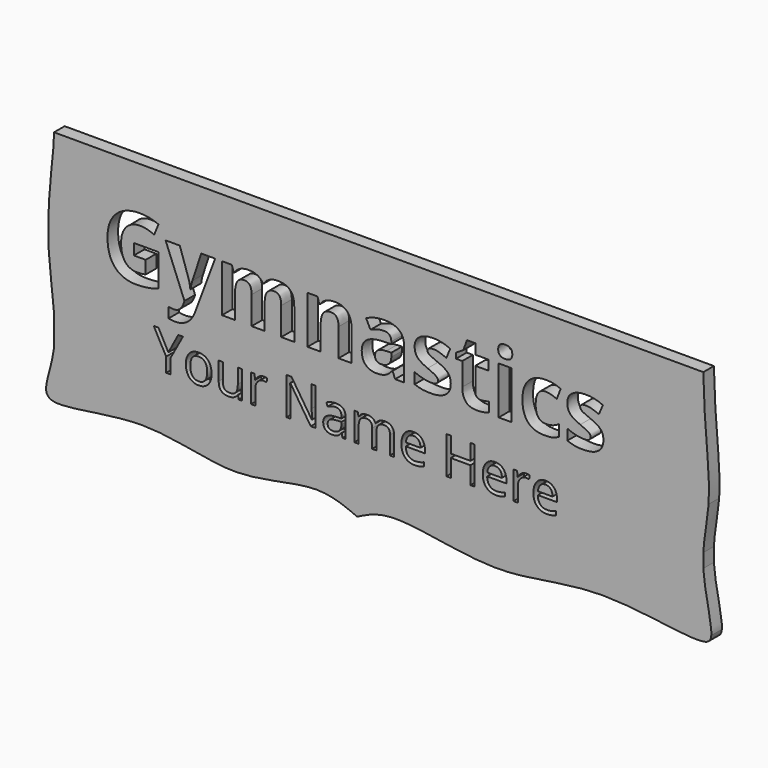
from build123d import *

# Parameters (mm, degrees)
F0_W         = 622.3
F0_H         = 219.71
F1_DEPTH     = 12.7
F2_TEXT_SIZE = 83.5725143433
F3_TEXT_SIZE = 50.0563092323
F4_DEPTH     = 25.4
F5_W         = 12.4444697139
F5_H         = 45.6253695493
F6_DEPTH     = 12.7


# Not quite as in the source:
# - Text() gives the source's letters only with a copy of the font that has no kerning and outlines rounded to 1/6400 em; it was checked with that copy


with BuildPart() as f1:
    # F0 (on Front) → F1 (new body)
    with BuildSketch(Plane.XZ):
        with Locations((20.5820777893, -3.9109852161)):
            Rectangle(F0_W, F0_H)
    extrude(amount=F1_DEPTH)

    # F2 (on face) + F3 (on face) → F4 (cut)
    with BuildSketch(Plane.XZ.offset(12.7)):
        with Locations((-244.2139566496, 3.9248836317)):
            Text('Gymnastics', F2_TEXT_SIZE, font='Open Sans', font_style=FontStyle.BOLD, text_align=(TextAlign.LEFT, TextAlign.BOTTOM))
    with BuildSketch(Plane.XZ.offset(12.7)):
        with Locations((-195.0602680445, -62.0602369308)):
            Text('Your Name Here', F3_TEXT_SIZE, font='Open Sans', text_align=(TextAlign.LEFT, TextAlign.BOTTOM))
    extrude(amount=-F4_DEPTH, mode=Mode.SUBTRACT)

    # F5 (on face) → F6 (join)
    with BuildSketch(Plane.XZ.offset(12.7)):
        with BuildLine():
            Line((0, -113.7659852161), (-38.9948076344, -113.7659852161))
            add(Edge.make_bspline(
                [(-38.9948076344, -113.7659852161), (-23.7077914674, -113.7998251226), (-11.8928807187, -118.8459366123), (0, -123.9259852161)],
                knots=[0.9046401261, 0.9046401261, 0.9046401261, 0.9046401261, 1, 1, 1, 1], degree=3))
            Line((0, -123.9259852161), (0, -113.7659852161))
        make_face()
        with BuildLine():
            Line((0, -113.7659852161), (0, -123.9259852161))
            add(Edge.make_bspline(
                [(33.4181897342, -113.7659852161), (18.7696313337, -114.397214566), (9.2754221357, -119.2324373573), (0, -123.9259852161)],
                knots=[0.9141845392, 0.9141845392, 0.9141845392, 0.9141845392, 1, 1, 1, 1], degree=3))
            Line((33.4181897343, -113.7659852161), (0, -113.7659852161))
        make_face()
        with BuildLine():
            Line((-115.3574213386, -113.7659852161), (-115.3574213386, -123.9259852161))
            add(Edge.make_bspline(
                [(-115.3574213386, -123.9259852161), (-88.4472145967, -123.5256265977), (-60.5272248515, -113.8129256595), (-39.3042191863, -113.7659852161)],
                knots=[0.7720146402, 0.7720146402, 0.7720146402, 0.7720146402, 0.9039977451, 0.9039977451, 0.9039977451, 0.9039977451], degree=3))
            Line((-39.3042191863, -113.7659852161), (-115.3574213386, -113.7659852161))
        make_face()
        with BuildLine():
            Line((-115.3574213386, -113.7659852161), (-205.5865424126, -113.7659852161))
            add(Edge.make_bspline(
                [(-205.5865424126, -113.7659852161), (-172.4059215865, -113.8913066112), (-144.4726963732, -124.3591499032), (-115.3574213386, -123.9259852161)],
                knots=[0.6292166144, 0.6292166144, 0.6292166144, 0.6292166144, 0.7720146402, 0.7720146402, 0.7720146402, 0.7720146402], degree=3))
            Line((-115.3574213386, -123.9259852161), (-115.3574213386, -113.7659852161))
        make_face()
        with BuildLine():
            Line((-206.7851424218, -113.7659852161), (-290.5679222107, -113.7659852161))
            Line((-290.5679222107, -113.7659852161), (-290.5679222107, -121.3859852161))
            add(Edge.make_bspline(
                [(-290.5679222107, -121.3859852161), (-276.2432745432, -123.9369942913), (-239.0205349915, -113.8882619563), (-206.7851424217, -113.7659852161)],
                knots=[0.4892995577, 0.4892995577, 0.4892995577, 0.4892995577, 0.6275004376, 0.6275004376, 0.6275004376, 0.6275004376], degree=3))
        make_face()
        with BuildLine():
            Line((-290.5679222107, -113.7659852161), (-298.1879222107, -113.7659852161))
            add(Edge.make_bspline(
                [(-298.1879222107, -113.7659852161), (-297.8884483653, -117.9460242514), (-295.6947312883, -120.4729759199), (-290.5679222107, -121.3859852161)],
                knots=[0.4398372922, 0.4398372922, 0.4398372922, 0.4398372922, 0.4892995577, 0.4892995577, 0.4892995577, 0.4892995577], degree=3))
            Line((-290.5679222107, -121.3859852161), (-290.5679222107, -113.7659852161))
        make_face()
        with BuildLine():
            Line((-290.5679222107, -113.7659852161), (-290.5679222107, -75.665985216))
            add(Edge.make_bspline(
                [(-290.5679222107, -75.6659852161), (-292.4954303089, -91.9313359206), (-298.7565718097, -105.8288062002), (-298.1879222107, -113.7659852161)],
                knots=[0.3459169119, 0.3459169119, 0.3459169119, 0.3459169119, 0.4398372922, 0.4398372922, 0.4398372922, 0.4398372922], degree=3))
            Line((-298.1879222107, -113.7659852161), (-290.5679222107, -113.7659852161))
        make_face()
        with BuildLine():
            Line((-290.5679222107, -46.9201377643), (-290.5679222107, 4.3440147839))
            Line((-290.5679222107, 4.3440147839), (-295.6479222107, 4.3440147839))
            add(Edge.make_bspline(
                [(-295.6479222107, 4.3440147839), (-294.6144050147, -13.1702112496), (-291.8699066313, -30.6290122267), (-290.5679222107, -46.9201377643)],
                knots=[0.2110057255, 0.2110057255, 0.2110057255, 0.2110057255, 0.2942177148, 0.2942177148, 0.2942177148, 0.2942177148], degree=3))
        make_face()
        with BuildLine():
            Line((-290.5679222107, 4.3440147839), (-290.5679222107, 74.1940147839))
            Line((-290.5679222107, 74.1940147839), (-293.1079222107, 74.1940147839))
            add(Edge.make_bspline(
                [(-293.1079222107, 74.1940147839), (-294.8560081938, 57.4984825083), (-297.212501225, 30.8577395787), (-295.6479222107, 4.3440147839)],
                knots=[0.0850361406, 0.0850361406, 0.0850361406, 0.0850361406, 0.2110057255, 0.2110057255, 0.2110057255, 0.2110057255], degree=3))
            Line((-295.6479222107, 4.3440147839), (-290.5679222107, 4.3440147839))
        make_face()
        with BuildLine():
            Line((-290.5679222107, 105.9440147839), (-290.5679222107, 74.1940147839))
            Line((-290.5679222107, 74.1940147839), (-290.5679222107, 4.3440147839))
            Line((-290.5679222107, 4.3440147839), (-290.5679222107, -46.9201377643))
            add(Edge.make_bspline(
                [(-290.5679222107, -46.9201377643), (-289.7590057341, -57.0417334302), (-289.5069105237, -66.7125975723), (-290.5679222107, -75.6659852161)],
                knots=[0.2942177148, 0.2942177148, 0.2942177148, 0.2942177148, 0.3459169119, 0.3459169119, 0.3459169119, 0.3459169119], degree=3))
            Line((-290.5679222107, -75.665985216), (-290.5679222107, -113.7659852161))
            Line((-290.5679222107, -113.7659852161), (-206.7851424218, -113.7659852161))
            add(Edge.make_bspline(
                [(-206.7851424217, -113.7659852161), (-206.3848437247, -113.764466785), (-205.9853141086, -113.7644790771), (-205.5865424126, -113.7659852161)],
                knots=[0.6275004376, 0.6275004376, 0.6275004376, 0.6275004376, 0.6292166144, 0.6292166144, 0.6292166144, 0.6292166144], degree=3))
            Line((-205.5865424126, -113.7659852161), (-115.3574213386, -113.7659852161))
            Line((-115.3574213386, -113.7659852161), (-39.3042191863, -113.7659852161))
            add(Edge.make_bspline(
                [(-39.3042191863, -113.7659852161), (-39.2009237185, -113.7657567501), (-39.0977868963, -113.7657572573), (-38.9948076344, -113.7659852161)],
                knots=[0.9039977451, 0.9039977451, 0.9039977451, 0.9039977451, 0.9046401261, 0.9046401261, 0.9046401261, 0.9046401261], degree=3))
            Line((-38.9948076344, -113.7659852161), (0, -113.7659852161))
            Line((0, -113.7659852161), (33.4181897343, -113.7659852161))
            add(Edge.make_bspline(
                [(40.8108736554, -113.7659852161), (38.2263464594, -113.671584288), (35.7565941218, -113.6652197045), (33.4181897342, -113.7659852161)],
                knots=[0.9004854949, 0.9004854949, 0.9004854949, 0.9004854949, 0.9141845392, 0.9141845392, 0.9141845392, 0.9141845392], degree=3))
            Line((40.8108736554, -113.7659852161), (131.6767185926, -113.7659852161))
            Line((131.6767185926, -113.7659852161), (234.9624951182, -113.7659852161))
            add(Edge.make_bspline(
                [(235.4865521193, -113.7659852161), (235.3117017675, -113.7657620078), (235.1370165153, -113.7657627033), (234.9624951182, -113.7659852161)],
                knots=[0.6215721476, 0.6215721476, 0.6215721476, 0.6215721476, 0.6222517313, 0.6222517313, 0.6222517313, 0.6222517313], degree=3))
            Line((235.4865521193, -113.7659852161), (331.7320777893, -113.7659852161))
            Line((331.7320777893, -113.7659852161), (331.7320777893, -59.7018413246))
            add(Edge.make_bspline(
                [(331.7320777893, -46.2929872824), (331.4882954863, -50.6263940713), (331.4498437355, -55.0775546721), (331.7320777893, -59.7018413246)],
                knots=[0.2992799759, 0.2992799759, 0.2992799759, 0.2992799759, 0.3239405291, 0.3239405291, 0.3239405291, 0.3239405291], degree=3))
            Line((331.7320777893, -46.2929872824), (331.7320777893, -3.9109852161))
            Line((331.7320777893, -3.9109852161), (331.7320777893, 54.1004016995))
            Line((331.7320777893, 54.1004016995), (331.7320777893, 105.9440147839))
            Line((331.7320777893, 105.9440147839), (-290.5679222107, 105.9440147839))
        make_face()
        Polygon((-190.516093722, -26.324724918), (-181.0523227578, -44.1963915736), (-171.525981407, -26.324724918), (-167.0287348744, -26.324724918), (-178.9562148086, -48.2008963122), (-178.9562148086, -62.0602369308), (-183.1562520052, -62.0602369308), (-183.1562520052, -48.3964287701), (-195.0602680445, -26.324724918), align=None, mode=Mode.SUBTRACT)
        with BuildLine():
            add(Edge.make_bspline(
                [(-139.6072629731, -48.6388890179), (-139.6072629731, -42.2645308891), (-146.231902648, -34.7795483993), (-157.6666407883, -34.7795483993), (-164.2208887784, -42.0924623262), (-164.2208887784, -52.8702114077), (-161.1862250312, -59.1741778517), (-155.6174606291, -62.5529787249), (-146.2006174548, -62.5529787249), (-139.6072629731, -55.193137008), (-139.6072629731, -48.6388890179)],
                knots=[0, 0, 0, 1, 2, 3.0362116992, 4.0724233983, 4.742185082, 5.4119467657, 6.0817084494, 7.1649751726, 8.2482418958, 8.2482418958, 8.2482418958], degree=2))
        make_face(mode=Mode.SUBTRACT)
        with BuildLine():
            Line((-132.7792695419, -35.2722901933), (-128.6730879252, -35.2722901933))
            Line((-128.6730879252, -35.2722901933), (-128.6730879252, -52.6512150548))
            add(Edge.make_bspline(
                [(-114.4305036889, -49.3506271648), (-114.4305036889, -54.5596118443), (-118.3098676544, -59.1507139567), (-125.6931732662, -59.1507139567), (-128.6730879252, -55.9283390499), (-128.6730879252, -52.6512150548)],
                knots=[0, 0, 0, 1, 2, 2.7546468401, 3.5092936803, 3.5092936803, 3.5092936803], degree=2))
            Line((-114.4305036889, -49.3506271648), (-114.4305036889, -35.2722901933))
            Line((-114.4305036889, -35.2722901933), (-110.3712498621, -35.2722901933))
            Line((-110.3712498621, -35.2722901933), (-110.3712498621, -62.0602369308))
            Line((-110.3712498621, -62.0602369308), (-113.718765542, -62.0602369308))
            Line((-113.718765542, -62.0602369308), (-114.3053629158, -58.4702610031))
            Line((-114.3053629158, -58.4702610031), (-114.5243592687, -58.4702610031))
            add(Edge.make_bspline(
                [(-132.7792695419, -52.7998197229), (-132.7792695419, -57.9071275242), (-127.9222432867, -62.5529787249), (-120.1948005489, -62.5529787249), (-115.7679457012, -60.4490494774), (-114.5243592687, -58.4702610031)],
                knots=[0, 0, 0, 1, 2, 2.5808, 3.1616, 3.1616, 3.1616], degree=2))
            Line((-132.7792695419, -52.7998197229), (-132.7792695419, -35.2722901933))
        make_face(mode=Mode.SUBTRACT)
        with BuildLine():
            add(Edge.make_bspline(
                [(-86.3442214306, -35.0767577353), (-87.7598764261, -34.7795483993), (-92.0615905007, -34.7795483993), (-96.2694489956, -37.6186796885), (-97.7554956759, -40.2309933266)],
                knots=[0, 0, 0, 1, 2.4122807018, 3.8245614035, 3.8245614035, 3.8245614035], degree=2))
            Line((-86.3442214306, -35.0767577353), (-86.9073549095, -38.8388022261))
            add(Edge.make_bspline(
                [(-97.708567886, -47.6846906232), (-97.708567886, -43.7505775695), (-93.0940018787, -38.4712012051), (-88.5654701528, -38.4712012051), (-86.9073549095, -38.8388022261)],
                knots=[0, 0, 0, 1, 2, 2.3918269231, 2.3918269231, 2.3918269231], degree=2))
            Line((-97.708567886, -47.6846906232), (-97.708567886, -62.0602369308))
            Line((-97.708567886, -62.0602369308), (-101.7678217128, -62.0602369308))
            Line((-101.7678217128, -62.0602369308), (-101.7678217128, -35.2722901933))
            Line((-101.7678217128, -35.2722901933), (-98.4203060329, -35.2722901933))
            Line((-98.4203060329, -35.2722901933), (-97.9510281338, -40.2309933266))
            Line((-97.9510281338, -40.2309933266), (-97.7554956759, -40.2309933266))
        make_face(mode=Mode.SUBTRACT)
        with BuildLine():
            Line((-11.1033316158, -62.0602369308), (-14.1145314681, -62.0602369308))
            Line((-14.1145314681, -62.0602369308), (-14.9201251948, -58.2434433519))
            Line((-14.9201251948, -58.2434433519), (-15.1156576527, -58.2434433519))
            add(Edge.make_bspline(
                [(-19.6129041853, -46.151716153), (-32.5884380941, -46.5427810688), (-32.5884380941, -58.4389758098), (-28.0677276666, -62.5529787249), (-21.0989508657, -62.5529787249), (-17.117910022, -60.7619014101), (-15.1156576527, -58.2434433519)],
                knots=[0, 0, 0, 1, 1.4667309547, 1.9334619094, 2.2837393645, 2.6340168197, 2.6340168197, 2.6340168197], degree=2))
            Line((-19.6129041853, -46.151716153), (-15.0687298628, -46.0031114849))
            Line((-15.0687298628, -46.0031114849), (-15.0687298628, -44.3371749433))
            add(Edge.make_bspline(
                [(-28.3336518094, -40.2309933266), (-24.1101507179, -38.1818131674), (-17.7748990807, -38.1818131674), (-15.0687298628, -41.1851917213), (-15.0687298628, -44.3371749433)],
                knots=[0, 0, 0, 1, 1.8925233645, 2.785046729, 2.785046729, 2.785046729], degree=2))
            Line((-28.3336518094, -40.2309933266), (-29.5850595402, -37.1259378945))
            add(Edge.make_bspline(
                [(-11.1033316158, -43.7740414644), (-11.1033316158, -39.0812624739), (-15.7257189215, -34.8342974875), (-22.8900281804, -34.8342974875), (-27.6062710659, -36.054420025), (-29.5850595402, -37.1259378945)],
                knots=[0, 0, 0, 1, 2, 2.4967320261, 2.9934640523, 2.9934640523, 2.9934640523], degree=2))
            Line((-11.1033316158, -43.7740414644), (-11.1033316158, -62.0602369308))
        make_face(mode=Mode.SUBTRACT)
        with BuildLine():
            Line((-67.7138888382, -26.324724918), (-63.0211098477, -26.324724918))
            Line((-63.0211098477, -26.324724918), (-43.5382557387, -56.1942631927))
            Line((-43.5382557387, -56.1942631927), (-43.3427232808, -56.1942631927))
            add(Edge.make_bspline(
                [(-43.6868604067, -46.8321691066), (-43.7337881966, -48.3729648751), (-43.3896510707, -55.537274134), (-43.3427232808, -56.1942631927)],
                knots=[0, 0, 0, 1, 2, 2, 2], degree=2))
            Line((-43.6868604067, -46.8321691066), (-43.6868604067, -26.324724918))
            Line((-43.6868604067, -26.324724918), (-39.7996751429, -26.324724918))
            Line((-39.7996751429, -26.324724918), (-39.7996751429, -62.0602369308))
            Line((-39.7996751429, -62.0602369308), (-44.5393819233, -62.0602369308))
            Line((-44.5393819233, -62.0602369308), (-64.0691638222, -32.0733791814))
            Line((-64.0691638222, -32.0733791814), (-64.2646962802, -32.0733791814))
            add(Edge.make_bspline(
                [(-64.2646962802, -32.0733791814), (-63.8736313643, -37.3527555457), (-63.8736313643, -41.7483252002)],
                knots=[0, 0, 0, 1, 1, 1], degree=2))
            Line((-63.8736313643, -41.7483252002), (-63.8736313643, -62.0602369308))
            Line((-63.8736313643, -62.0602369308), (-67.7138888382, -62.0602369308))
            Line((-67.7138888382, -62.0602369308), (-67.7138888382, -26.324724918))
        make_face(mode=Mode.SUBTRACT)
        with BuildLine():
            Line((35.4490359702, -62.0602369308), (31.3976034417, -62.0602369308))
            Line((31.3976034417, -62.0602369308), (31.3976034417, -44.6343842794))
            add(Edge.make_bspline(
                [(18.3673204447, -47.0980932494), (18.3673204447, -42.5773828218), (21.9885815657, -38.2287409573), (28.6601490306, -38.2287409573), (31.3976034417, -41.4276519692), (31.3976034417, -44.6343842794)],
                knots=[0, 0, 0, 1, 2, 2.7623966942, 3.5247933884, 3.5247933884, 3.5247933884], degree=2))
            Line((18.3673204447, -47.0980932494), (18.3673204447, -62.0602369308))
            Line((18.3673204447, -62.0602369308), (14.3080666179, -62.0602369308))
            Line((14.3080666179, -62.0602369308), (14.3080666179, -44.6343842794))
            add(Edge.make_bspline(
                [(1.3090688141, -48.0053638542), (1.3090688141, -42.7963791747), (4.852116952, -38.2287409573), (11.5706122067, -38.2287409573), (14.3080666179, -41.4276519692), (14.3080666179, -44.6343842794)],
                knots=[0, 0, 0, 1, 2, 2.7638603696, 3.5277207392, 3.5277207392, 3.5277207392], degree=2))
            Line((1.3090688141, -48.0053638542), (1.3090688141, -62.0602369308))
            Line((1.3090688141, -62.0602369308), (-2.7501850127, -62.0602369308))
            Line((-2.7501850127, -62.0602369308), (-2.7501850127, -35.2722901933))
            Line((-2.7501850127, -35.2722901933), (0.5504028773, -35.2722901933))
            Line((0.5504028773, -35.2722901933), (1.207391936, -38.9404791042))
            Line((1.207391936, -38.9404791042), (1.4029243939, -38.9404791042))
            add(Edge.make_bspline(
                [(17.538262823, -39.3315440201), (15.6064021386, -34.7795483993), (6.7370498465, -34.7795483993), (2.5526552466, -36.9851545248), (1.4029243939, -38.9404791042)],
                knots=[0, 0, 0, 1, 1.4122042341, 1.8244084682, 1.8244084682, 1.8244084682], degree=2))
            Line((17.538262823, -39.3315440201), (17.7337952809, -39.3315440201))
            add(Edge.make_bspline(
                [(35.4490359702, -44.5874564895), (35.4490359702, -39.4488634948), (30.9283255426, -34.7795483993), (23.474628246, -34.7795483993), (18.9304539235, -37.2276147726), (17.7337952809, -39.3315440201)],
                knots=[0, 0, 0, 1, 2, 2.6402753873, 3.2805507745, 3.2805507745, 3.2805507745], degree=2))
            Line((35.4490359702, -44.5874564895), (35.4490359702, -62.0602369308))
        make_face(mode=Mode.SUBTRACT)
        with BuildLine():
            add(Edge.make_bspline(
                [(64.9744371189, -46.8321691066), (64.9744371189, -41.4041880742), (59.1084633808, -34.7795483993), (48.6983153201, -34.7795483993), (42.316135893, -42.4053142589), (42.316135893, -55.3104564828), (49.1910571141, -62.5529787249), (57.8414130533, -62.5529787249), (61.6738492289, -61.7395636998), (63.8247062662, -60.8166504984)],
                knots=[0, 0, 0, 1, 2, 3.0699844479, 4.1399688958, 5.1996278002, 6.2592867045, 6.743742093, 7.2281974814, 7.2281974814, 7.2281974814], degree=2))
            Line((64.9744371189, -46.8321691066), (64.9744371189, -49.3975549547))
            Line((64.9744371189, -49.3975549547), (46.5239943878, -49.3975549547))
            add(Edge.make_bspline(
                [(63.8247062662, -57.1953893773), (59.6012051748, -59.0021092887), (51.1698455884, -59.0021092887), (46.6491351609, -54.1137978402), (46.5239943878, -49.3975549547)],
                knots=[0, 0, 0, 1, 1.9493670886, 2.8987341772, 2.8987341772, 2.8987341772], degree=2))
            Line((63.8247062662, -57.1953893773), (63.8247062662, -60.8166504984))
        make_face(mode=Mode.SUBTRACT)
        Polygon((112.6452503643, -26.324724918), (112.6452503643, -62.0602369308), (108.4921409577, -62.0602369308), (108.4921409577, -45.2444455481), (89.6662759074, -45.2444455481), (89.6662759074, -62.0602369308), (85.5131665008, -62.0602369308), (85.5131665008, -26.324724918), (89.6662759074, -26.324724918), (89.6662759074, -41.5293288473), (108.4921409577, -41.5293288473), (108.4921409577, -26.324724918), align=None, mode=Mode.SUBTRACT)
        with BuildLine():
            add(Edge.make_bspline(
                [(142.9997091347, -46.8321691066), (142.9997091347, -41.4041880742), (137.1337353966, -34.7795483993), (126.7235873359, -34.7795483993), (120.3414079088, -42.4053142589), (120.3414079088, -55.3104564828), (127.2163291299, -62.5529787249), (135.8666850691, -62.5529787249), (139.6991212447, -61.7395636998), (141.8499782821, -60.8166504984)],
                knots=[0, 0, 0, 1, 2, 3.0699844479, 4.1399688958, 5.1996278002, 6.2592867045, 6.743742093, 7.2281974814, 7.2281974814, 7.2281974814], degree=2))
            Line((142.9997091347, -46.8321691066), (142.9997091347, -49.3975549547))
            Line((142.9997091347, -49.3975549547), (124.5492664036, -49.3975549547))
            add(Edge.make_bspline(
                [(141.8499782821, -57.1953893773), (137.6264771906, -59.0021092887), (129.1951176043, -59.0021092887), (124.6744071767, -54.1137978402), (124.5492664036, -49.3975549547)],
                knots=[0, 0, 0, 1, 1.9493670886, 2.8987341772, 2.8987341772, 2.8987341772], degree=2))
            Line((141.8499782821, -57.1953893773), (141.8499782821, -60.8166504984))
        make_face(mode=Mode.SUBTRACT)
        with BuildLine():
            add(Edge.make_bspline(
                [(165.345158428, -35.0767577353), (163.9295034325, -34.7795483993), (159.6277893578, -34.7795483993), (155.419930863, -37.6186796885), (153.9338841827, -40.2309933266)],
                knots=[0, 0, 0, 1, 2.4122807018, 3.8245614035, 3.8245614035, 3.8245614035], degree=2))
            Line((165.345158428, -35.0767577353), (164.7820249491, -38.8388022261))
            add(Edge.make_bspline(
                [(153.9808119726, -47.6846906232), (153.9808119726, -43.7505775695), (158.5953779799, -38.4712012051), (163.1239097058, -38.4712012051), (164.7820249491, -38.8388022261)],
                knots=[0, 0, 0, 1, 2, 2.3918269231, 2.3918269231, 2.3918269231], degree=2))
            Line((153.9808119726, -47.6846906232), (153.9808119726, -62.0602369308))
            Line((153.9808119726, -62.0602369308), (149.9215581458, -62.0602369308))
            Line((149.9215581458, -62.0602369308), (149.9215581458, -35.2722901933))
            Line((149.9215581458, -35.2722901933), (153.2690738257, -35.2722901933))
            Line((153.2690738257, -35.2722901933), (153.7383517247, -40.2309933266))
            Line((153.7383517247, -40.2309933266), (153.9338841827, -40.2309933266))
        make_face(mode=Mode.SUBTRACT)
        with BuildLine():
            add(Edge.make_bspline(
                [(191.5230438968, -46.8321691066), (191.5230438968, -41.4041880742), (185.6570701586, -34.7795483993), (175.246922098, -34.7795483993), (168.8647426708, -42.4053142589), (168.8647426708, -55.3104564828), (175.739663892, -62.5529787249), (184.3900198312, -62.5529787249), (188.2224560068, -61.7395636998), (190.3733130441, -60.8166504984)],
                knots=[0, 0, 0, 1, 2, 3.0699844479, 4.1399688958, 5.1996278002, 6.2592867045, 6.743742093, 7.2281974814, 7.2281974814, 7.2281974814], degree=2))
            Line((191.5230438968, -46.8321691066), (191.5230438968, -49.3975549547))
            Line((191.5230438968, -49.3975549547), (173.0726011657, -49.3975549547))
            add(Edge.make_bspline(
                [(190.3733130441, -57.1953893773), (186.1498119526, -59.0021092887), (177.7184523663, -59.0021092887), (173.1977419388, -54.1137978402), (173.0726011657, -49.3975549547)],
                knots=[0, 0, 0, 1, 1.9493670886, 2.8987341772, 2.8987341772, 2.8987341772], degree=2))
            Line((190.3733130441, -57.1953893773), (190.3733130441, -60.8166504984))
        make_face(mode=Mode.SUBTRACT)
        with BuildLine():
            Line((-149.502793129, 49.550253181), (-136.1573072448, 49.550253181))
            Line((-136.1573072448, 49.550253181), (-155.457334776, -1.9121341669))
            add(Edge.make_bspline(
                [(-180.8424860078, -15.4534931316), (-177.747691336, -16.1586362214), (-167.9540373114, -16.1586362214), (-158.1212086707, -9.0549725022), (-155.457334776, -1.9121341669)],
                knots=[0, 0, 0, 1, 3.036437247, 5.0728744939, 5.0728744939, 5.0728744939], degree=2))
            Line((-180.8424860078, -15.4534931316), (-180.8424860078, -5.5814898748))
            add(Edge.make_bspline(
                [(-166.3217616406, 2.0053274429), (-167.7059314094, -2.0688326313), (-172.6419330378, -6.1168762948), (-178.5964746848, -6.1168762948), (-180.8424860078, -5.5814898748)],
                knots=[0, 0, 0, 1, 2, 2.8023715415, 2.8023715415, 2.8023715415], degree=2))
            Line((-166.3217616406, 2.0053274429), (-165.5774439347, 4.2513387659))
            Line((-165.5774439347, 4.2513387659), (-183.7022329829, 49.550253181))
            Line((-183.7022329829, 49.550253181), (-170.0694665807, 49.550253181))
            Line((-170.0694665807, 49.550253181), (-161.4641092444, 23.8778214312))
            add(Edge.make_bspline(
                [(-161.4641092444, 23.8778214312), (-160.3541617883, 20.5349208575), (-159.9493574219, 15.9645489793)],
                knots=[0, 0, 0, 1, 1, 1], degree=2))
            Line((-159.9493574219, 15.9645489793), (-159.70125152, 15.9645489793))
            add(Edge.make_bspline(
                [(-159.70125152, 15.9645489793), (-159.2572725375, 20.1692911072), (-157.9514520009, 23.8778214312)],
                knots=[0, 0, 0, 1, 1, 1], degree=2))
            Line((-157.9514520009, 23.8778214312), (-149.502793129, 49.550253181))
        make_face(mode=Mode.SUBTRACT)
        with BuildLine():
            Line((-214.0625604592, 37.4322386012), (-190.3880341304, 37.4322386012))
            Line((-190.3880341304, 37.4322386012), (-190.3880341304, 6.4973500889))
            add(Edge.make_bspline(
                [(-190.4663833626, 60.7672515905), (-198.9933914667, 64.4366072984), (-222.8246162599, 64.4366072984), (-239.3563042534, 48.2836072605), (-239.3563042534, 18.9809944189), (-225.109802199, 3.1022166937), (-206.3059864717, 3.1022166937), (-196.1467026969, 4.6169685161), (-190.3880341304, 6.4973500889)],
                knots=[0, 0, 0, 1, 2.5923295455, 4.1846590909, 5.823059654, 7.461460217, 8.1047780396, 8.7480958623, 8.7480958623, 8.7480958623], degree=2))
            Line((-190.4663833626, 60.7672515905), (-194.6711254905, 50.6471424318))
            add(Edge.make_bspline(
                [(-202.7541546121, 14.4497971568), (-206.8283146864, 13.6401884241), (-218.3848264354, 13.6401884241), (-226.3372735034, 23.8778214312), (-226.3372735034, 42.8905684443), (-216.4652702466, 53.9116937733), (-201.2002281736, 53.9116937733), (-194.6711254905, 50.6471424318)],
                knots=[0, 0, 0, 1, 2.9111842105, 4.8223684211, 6.6513511602, 8.4803338993, 10.0559384564, 10.0559384564, 10.0559384564], degree=2))
            Line((-202.7541546121, 14.4497971568), (-202.7541546121, 26.8942668708))
            Line((-202.7541546121, 26.8942668708), (-214.0625604592, 26.8942668708))
            Line((-214.0625604592, 26.8942668708), (-214.0625604592, 37.4322386012))
        make_face(mode=Mode.SUBTRACT)
        with BuildLine():
            add(Edge.make_bspline(
                [(-117.1837348478, 25.3925732537), (-117.1837348478, 33.4233695538), (-112.8614688717, 40.4486840408), (-104.5303338481, 40.4486840408), (-101.2266078904, 35.5126824124), (-101.2266078904, 30.576680784)],
                knots=[0, 0, 0, 1, 2, 2.7431693989, 3.4863387978, 3.4863387978, 3.4863387978], degree=2))
            Line((-117.1837348478, 25.3925732537), (-117.1837348478, 3.9248836317))
            Line((-117.1837348478, 3.9248836317), (-129.6282045618, 3.9248836317))
            Line((-129.6282045618, 3.9248836317), (-129.6282045618, 49.550253181))
            Line((-129.6282045618, 49.550253181), (-120.1218310552, 49.550253181))
            Line((-120.1218310552, 49.550253181), (-118.4503807684, 43.7132353824))
            Line((-118.4503807684, 43.7132353824), (-117.758295884, 43.7132353824))
            add(Edge.make_bspline(
                [(-90.6102869278, 43.7132353824), (-94.2535262249, 50.3990365298), (-108.9831818779, 50.3990365298), (-115.9170889273, 46.8602628756), (-117.758295884, 43.7132353824)],
                knots=[0, 0, 0, 1, 1.4387755102, 1.8775510204, 1.8775510204, 1.8775510204], degree=2))
            Line((-90.6102869278, 43.7132353824), (-89.513397677, 43.7132353824))
            add(Edge.make_bspline(
                [(-60.3413668891, 33.6714754558), (-60.3413668891, 42.4465894618), (-68.293813957, 50.3990365298), (-80.5424105905, 50.3990365298), (-87.6721907204, 46.8994374917), (-89.513397677, 43.7132353824)],
                knots=[0, 0, 0, 1, 2, 2.5791245791, 3.1582491582, 3.1582491582, 3.1582491582], degree=2))
            Line((-60.3413668891, 33.6714754558), (-60.3413668891, 3.9248836317))
            Line((-60.3413668891, 3.9248836317), (-72.8250112191, 3.9248836317))
            Line((-72.8250112191, 3.9248836317), (-72.8250112191, 30.576680784))
            add(Edge.make_bspline(
                [(-88.7821381765, 26.8159176386), (-88.7821381765, 33.9195813578), (-84.2509409145, 40.4486840408), (-76.1287371767, 40.4486840408), (-72.8250112191, 35.5126824124), (-72.8250112191, 30.576680784)],
                knots=[0, 0, 0, 1, 2, 2.7771428571, 3.5542857143, 3.5542857143, 3.5542857143], degree=2))
            Line((-88.7821381765, 26.8159176386), (-88.7821381765, 3.9248836317))
            Line((-88.7821381765, 3.9248836317), (-101.2266078904, 3.9248836317))
            Line((-101.2266078904, 3.9248836317), (-101.2266078904, 30.576680784))
        make_face(mode=Mode.SUBTRACT)
        with BuildLine():
            Line((-5.4577297352, 3.9248836317), (-17.9021994491, 3.9248836317))
            Line((-17.9021994491, 3.9248836317), (-17.9021994491, 30.576680784))
            add(Edge.make_bspline(
                [(-35.125972327, 25.3925732537), (-35.125972327, 33.4756023753), (-30.4772512167, 40.4486840408), (-21.4148566926, 40.4486840408), (-17.9021994491, 35.5126824124), (-17.9021994491, 30.576680784)],
                knots=[0, 0, 0, 1, 2, 2.735, 3.47, 3.47, 3.47], degree=2))
            Line((-35.125972327, 25.3925732537), (-35.125972327, 3.9248836317))
            Line((-35.125972327, 3.9248836317), (-47.570442041, 3.9248836317))
            Line((-47.570442041, 3.9248836317), (-47.570442041, 49.550253181))
            Line((-47.570442041, 49.550253181), (-38.0640685344, 49.550253181))
            Line((-38.0640685344, 49.550253181), (-36.3926182476, 43.7132353824))
            Line((-36.3926182476, 43.7132353824), (-35.7005333632, 43.7132353824))
            add(Edge.make_bspline(
                [(-5.4577297352, 33.6714754558), (-5.4577297352, 41.7936791935), (-13.6974573212, 50.3990365298), (-26.3116837049, 50.3990365298), (-33.6112205046, 47.01696134), (-35.7005333632, 43.7132353824)],
                knots=[0, 0, 0, 1, 2, 2.5836065574, 3.1672131148, 3.1672131148, 3.1672131148], degree=2))
            Line((-5.4577297352, 33.6714754558), (-5.4577297352, 3.9248836317))
        make_face(mode=Mode.SUBTRACT)
        with BuildLine():
            Line((36.3285274364, 3.9248836317), (33.9127594437, 10.1275311807))
            Line((33.9127594437, 10.1275311807), (33.5863043096, 10.1275311807))
            add(Edge.make_bspline(
                [(24.7328410713, 32.0783744011), (14.4952080643, 31.7127446509), (4.3359242894, 24.8180122176), (4.3359242894, 10.6237429846), (11.883566991, 3.1022166937), (23.792650285, 3.1022166937), (30.4523350217, 6.1708949547), (33.5863043096, 10.1275311807)],
                knots=[0, 0, 0, 1, 2, 2.9550359712, 3.9100719424, 4.6866320065, 5.4631920706, 5.4631920706, 5.4631920706], degree=2))
            Line((24.7328410713, 32.0783744011), (32.6591717286, 32.3264803031))
            Line((32.6591717286, 32.3264803031), (32.6591717286, 34.3243857241))
            add(Edge.make_bspline(
                [(12.6931757237, 37.9545668159), (20.084119961, 41.2582927735), (32.6591717286, 41.2582927735), (32.6591717286, 34.3243857241)],
                knots=[0, 0, 0, 1, 2.2983293556, 2.2983293556, 2.2983293556], degree=2))
            Line((12.6931757237, 37.9545668159), (8.5798410334, 46.3640510717))
            add(Edge.make_bspline(
                [(45.0122340049, 34.3243857241), (45.0122340049, 42.4857640779), (35.2185799803, 50.4904439674), (16.4539388692, 50.4904439674), (8.5798410334, 46.3640510717)],
                knots=[0, 0, 0, 1, 2, 3.0440967283, 3.0440967283, 3.0440967283], degree=2))
            Line((45.0122340049, 34.3243857241), (45.0122340049, 3.9248836317))
            Line((45.0122340049, 3.9248836317), (36.3285274364, 3.9248836317))
        make_face(mode=Mode.SUBTRACT)
        with BuildLine():
            add(Edge.make_bspline(
                [(55.145401369, 5.7660905884), (58.2010214247, 4.4602700518), (65.2263359117, 3.1022166937), (79.9168169486, 3.1022166937), (89.6712963571, 10.4539863148), (89.6712963571, 20.8613759916), (87.2947029805, 25.7582030039), (82.319526736, 29.505907944), (76.9787207412, 31.6735700348)],
                knots=[0, 0, 0, 1, 2, 3.9527559055, 5.905511811, 6.8455931856, 7.7856745602, 8.7257559348, 8.7257559348, 8.7257559348], degree=2))
            Line((55.145401369, 5.7660905884), (55.145401369, 16.0428982115))
            add(Edge.make_bspline(
                [(67.5115218508, 23.3032603951), (71.1808775587, 21.7623921619), (75.581492767, 19.4380316067), (77.3835251076, 17.5968246501), (77.3835251076, 12.2037858339), (67.3025905649, 12.2037858339), (58.6058257911, 14.4106225408), (55.145401369, 16.0428982115)],
                knots=[0, 0, 0, 1, 2, 3, 5.6548672566, 6.9490511024, 8.2432349481, 8.2432349481, 8.2432349481], degree=2))
            add(Edge.make_bspline(
                [(89.1750845532, 46.8080300541), (81.3793359496, 50.3990365298), (64.4820182058, 50.3990365298), (55.0670521368, 43.7524099985), (55.0670521368, 34.1285126436), (57.3000052545, 29.2708602474), (62.2490650882, 25.510097102), (67.5115218508, 23.3032603951)],
                knots=[0, 0, 0, 1, 2.0507131537, 3.1014263074, 3.7124633561, 4.3235004047, 4.9345374533, 4.9345374533, 4.9345374533], degree=2))
            Line((89.1750845532, 46.8080300541), (85.4273796131, 37.8370429676))
            add(Edge.make_bspline(
                [(76.9787207412, 31.6735700348), (70.9719462728, 34.0762798222), (67.4201144132, 36.531222431), (67.4201144132, 41.1799435413), (76.0385299549, 41.1799435413), (81.9930716018, 39.2995619686), (85.4273796131, 37.8370429676)],
                knots=[0, 0, 0, 1, 2, 3.78125, 4.7858412322, 5.7904324645, 5.7904324645, 5.7904324645], degree=2))
        make_face(mode=Mode.SUBTRACT)
        with BuildLine():
            add(Edge.make_bspline(
                [(126.4301444628, 14.4497971568), (121.8597725846, 13.0264527719), (116.1402786343, 13.0264527719), (113.1630078108, 15.559744613), (113.1630078108, 18.2105603023)],
                knots=[0, 0, 0, 1, 1.752, 2.504, 2.504, 2.504], degree=2))
            Line((126.4301444628, 14.4497971568), (126.4301444628, 5.1915295523))
            add(Edge.make_bspline(
                [(100.7185380969, 18.2105603023), (100.7185380969, 10.6629176007), (107.534921298, 3.1022166937), (121.7814233524, 3.1022166937), (126.4301444628, 5.1915295523)],
                knots=[0, 0, 0, 1, 2, 2.9073426573, 2.9073426573, 2.9073426573], degree=2))
            Line((100.7185380969, 18.2105603023), (100.7185380969, 40.2005781389))
            Line((100.7185380969, 40.2005781389), (94.7639964499, 40.2005781389))
            Line((94.7639964499, 40.2005781389), (94.7639964499, 45.4630349014))
            Line((94.7639964499, 45.4630349014), (101.6195542671, 49.6286024132))
            Line((101.6195542671, 49.6286024132), (105.2105607428, 59.2655579734))
            Line((105.2105607428, 59.2655579734), (113.1630078108, 59.2655579734))
            Line((113.1630078108, 59.2655579734), (113.1630078108, 49.550253181))
            Line((113.1630078108, 49.550253181), (125.9339326589, 49.550253181))
            Line((125.9339326589, 49.550253181), (125.9339326589, 40.2005781389))
            Line((125.9339326589, 40.2005781389), (113.1630078108, 40.2005781389))
            Line((113.1630078108, 40.2005781389), (113.1630078108, 18.2105603023))
        make_face(mode=Mode.SUBTRACT)
        with Locations((141.8714723082, 26.7375684064)):
            Rectangle(F5_W, F5_H, mode=Mode.SUBTRACT)
        with BuildLine():
            add(Edge.make_bspline(
                [(194.985722635, 47.304241858), (188.6916676485, 50.3990365298), (169.9662011535, 50.3990365298), (158.3835729937, 38.1243234857), (158.3835729937, 3.1022166937), (184.3694016723, 3.1022166937), (190.5328746051, 4.5777939001), (193.5493200447, 6.4973500889)],
                knots=[0, 0, 0, 1, 2.3663366337, 3.7326732673, 6.4791479148, 7.083675443, 7.6882029711, 7.6882029711, 7.6882029711], degree=2))
            Line((194.985722635, 47.304241858), (191.3033087217, 37.6672862978))
            add(Edge.make_bspline(
                [(193.5493200447, 17.1528456676), (190.493699989, 15.1027074252), (184.3694016723, 13.1831512363), (171.0630904042, 13.1831512363), (171.0630904042, 40.3703348086), (183.3116870377, 40.3703348086), (188.3652125144, 38.8555829862), (191.3033087217, 37.6672862978)],
                knots=[0, 0, 0, 1, 2, 4.7054545455, 7.4953720621, 8.2228505543, 8.9503290466, 8.9503290466, 8.9503290466], degree=2))
            Line((193.5493200447, 17.1528456676), (193.5493200447, 6.4973500889))
        make_face(mode=Mode.SUBTRACT)
        with BuildLine():
            add(Edge.make_bspline(
                [(201.4364760859, 5.7660905884), (204.4920961415, 4.4602700518), (211.5174106285, 3.1022166937), (226.2078916654, 3.1022166937), (235.9623710739, 10.4539863148), (235.9623710739, 20.8613759916), (233.5857776973, 25.7582030039), (228.6106014528, 29.505907944), (223.269795458, 31.6735700348)],
                knots=[0, 0, 0, 1, 2, 3.9527559055, 5.905511811, 6.8455931856, 7.7856745602, 8.7257559348, 8.7257559348, 8.7257559348], degree=2))
            Line((201.4364760859, 5.7660905884), (201.4364760859, 16.0428982115))
            add(Edge.make_bspline(
                [(213.8025965676, 23.3032603951), (217.4719522755, 21.7623921619), (221.8725674839, 19.4380316067), (223.6745998244, 17.5968246501), (223.6745998244, 12.2037858339), (213.5936652817, 12.2037858339), (204.8969005079, 14.4106225408), (201.4364760859, 16.0428982115)],
                knots=[0, 0, 0, 1, 2, 3, 5.6548672566, 6.9490511024, 8.2432349481, 8.2432349481, 8.2432349481], degree=2))
            add(Edge.make_bspline(
                [(235.46615927, 46.8080300541), (227.6704106664, 50.3990365298), (210.7730929226, 50.3990365298), (201.3581268537, 43.7524099985), (201.3581268537, 34.1285126436), (203.5910799713, 29.2708602474), (208.540139805, 25.510097102), (213.8025965676, 23.3032603951)],
                knots=[0, 0, 0, 1, 2.0507131537, 3.1014263074, 3.7124633561, 4.3235004047, 4.9345374533, 4.9345374533, 4.9345374533], degree=2))
            Line((235.46615927, 46.8080300541), (231.7184543299, 37.8370429676))
            add(Edge.make_bspline(
                [(223.269795458, 31.6735700348), (217.2630209896, 34.0762798222), (213.71118913, 36.531222431), (213.71118913, 41.1799435413), (222.3296046717, 41.1799435413), (228.2841463186, 39.2995619686), (231.7184543299, 37.8370429676)],
                knots=[0, 0, 0, 1, 2, 3.78125, 4.7858412322, 5.7904324645, 5.7904324645, 5.7904324645], degree=2))
        make_face(mode=Mode.SUBTRACT)
        with BuildLine():
            add(Edge.make_bspline(
                [(135.1138510313, 61.3418126266), (135.1138510313, 55.2175143099), (145.2861930115, 55.2175143099), (148.6682682013, 58.4428910354), (148.6682682013, 67.4269363273), (135.1138510313, 67.4269363273), (135.1138510313, 61.3418126266)],
                knots=[0, 0, 0, 1, 1.5009633911, 2.0019267823, 3.0534985853, 4.1050703883, 4.1050703883, 4.1050703883], degree=2))
        make_face(mode=Mode.SUBTRACT)
        with BuildLine():
            add(Edge.make_bspline(
                [(131.6767185926, -123.9259852161), (100.5310061435, -123.5697120198), (65.4537440273, -114.6660762799), (40.8108736554, -113.7659852161)],
                knots=[0.7698682692, 0.7698682692, 0.7698682692, 0.7698682692, 0.9004854949, 0.9004854949, 0.9004854949, 0.9004854949], degree=3))
            Line((131.6767185926, -123.9259852161), (131.6767185926, -113.7659852161))
            Line((131.6767185926, -113.7659852161), (40.8108736554, -113.7659852161))
        make_face()
        with BuildLine():
            add(Edge.make_bspline(
                [(234.9624951182, -113.7659852161), (197.0536312733, -113.8143185843), (166.8759215788, -124.3286259511), (131.6767185926, -123.9259852161)],
                knots=[0.6222517313, 0.6222517313, 0.6222517313, 0.6222517313, 0.7698682692, 0.7698682692, 0.7698682692, 0.7698682692], degree=3))
            Line((234.9624951182, -113.7659852161), (131.6767185926, -113.7659852161))
            Line((131.6767185926, -113.7659852161), (131.6767185926, -123.9259852161))
        make_face()
        with BuildLine():
            Line((331.7320777893, -121.3859852161), (331.7320777893, -113.7659852161))
            Line((331.7320777893, -113.7659852161), (235.4865521193, -113.7659852161))
            add(Edge.make_bspline(
                [(331.7320777893, -121.3859852161), (316.1806784758, -123.7284956134), (272.1951498612, -113.8128462119), (235.4865521193, -113.7659852161)],
                knots=[0.4788983528, 0.4788983528, 0.4788983528, 0.4788983528, 0.6215721476, 0.6215721476, 0.6215721476, 0.6215721476], degree=3))
        make_face()
        with BuildLine():
            add(Edge.make_bspline(
                [(339.3520777893, -113.7659852161), (338.9495303159, -118.4525306772), (336.9276781302, -120.6033708948), (331.7320777893, -121.3859852161)],
                knots=[0.4312321588, 0.4312321588, 0.4312321588, 0.4312321588, 0.4788983528, 0.4788983528, 0.4788983528, 0.4788983528], degree=3))
            Line((339.3520777893, -113.7659852161), (331.7320777893, -113.7659852161))
            Line((331.7320777893, -113.7659852161), (331.7320777893, -121.3859852161))
        make_face()
        with BuildLine():
            add(Edge.make_bspline(
                [(331.7320777893, -59.7018413246), (332.9600044823, -79.8209054161), (340.2581701542, -103.2170603302), (339.3520777893, -113.7659852161)],
                knots=[0.3239405291, 0.3239405291, 0.3239405291, 0.3239405291, 0.4312321588, 0.4312321588, 0.4312321588, 0.4312321588], degree=3))
            Line((331.7320777893, -59.7018413246), (331.7320777893, -113.7659852161))
            Line((331.7320777893, -113.7659852161), (339.3520777893, -113.7659852161))
        make_face()
        with BuildLine():
            add(Edge.make_bspline(
                [(336.8120777893, -3.9109852161), (335.7767608867, -18.131391827), (332.5626628965, -31.5287361559), (331.7320777893, -46.2929872824)],
                knots=[0.2152595692, 0.2152595692, 0.2152595692, 0.2152595692, 0.2992799759, 0.2992799759, 0.2992799759, 0.2992799759], degree=3))
            Line((336.8120777893, -3.9109852161), (331.7320777893, -3.9109852161))
            Line((331.7320777893, -3.9109852161), (331.7320777893, -46.2929872824))
        make_face()
        with BuildLine():
            add(Edge.make_bspline(
                [(334.2720777893, 54.1004016995), (335.7603698578, 34.9703279681), (338.175494417, 14.8159753674), (336.8120777893, -3.9109852161)],
                knots=[0.1046124627, 0.1046124627, 0.1046124627, 0.1046124627, 0.2152595692, 0.2152595692, 0.2152595692, 0.2152595692], degree=3))
            Line((334.2720777893, 54.1004016995), (331.7320777893, 54.1004016995))
            Line((331.7320777893, 54.1004016995), (331.7320777893, -3.9109852161))
            Line((331.7320777893, -3.9109852161), (336.8120777893, -3.9109852161))
        make_face()
        with BuildLine():
            add(Edge.make_bspline(
                [(331.7320777893, 105.9440147839), (332.2863265746, 89.3582595561), (332.8649565065, 72.1871297407), (334.2720777893, 54.1004016995)],
                knots=[0, 0, 0, 0, 0.1046124627, 0.1046124627, 0.1046124627, 0.1046124627], degree=3))
            Line((331.7320777893, 105.9440147839), (331.7320777893, 54.1004016995))
            Line((331.7320777893, 54.1004016995), (334.2720777893, 54.1004016995))
        make_face()
        with BuildLine():
            Line((-293.1079222107, 74.1940147839), (-290.5679222107, 74.1940147839))
            Line((-290.5679222107, 74.1940147839), (-290.5679222107, 105.9440147839))
            add(Edge.make_bspline(
                [(-290.5679222107, 105.9440147839), (-291.02506995, 92.2027539823), (-291.9278716013, 85.4643831904), (-293.1079222107, 74.1940147839)],
                knots=[0, 0, 0, 0, 0.0850361406, 0.0850361406, 0.0850361406, 0.0850361406], degree=3))
        make_face()
    extrude(amount=-F6_DEPTH)


solid = f1.part
